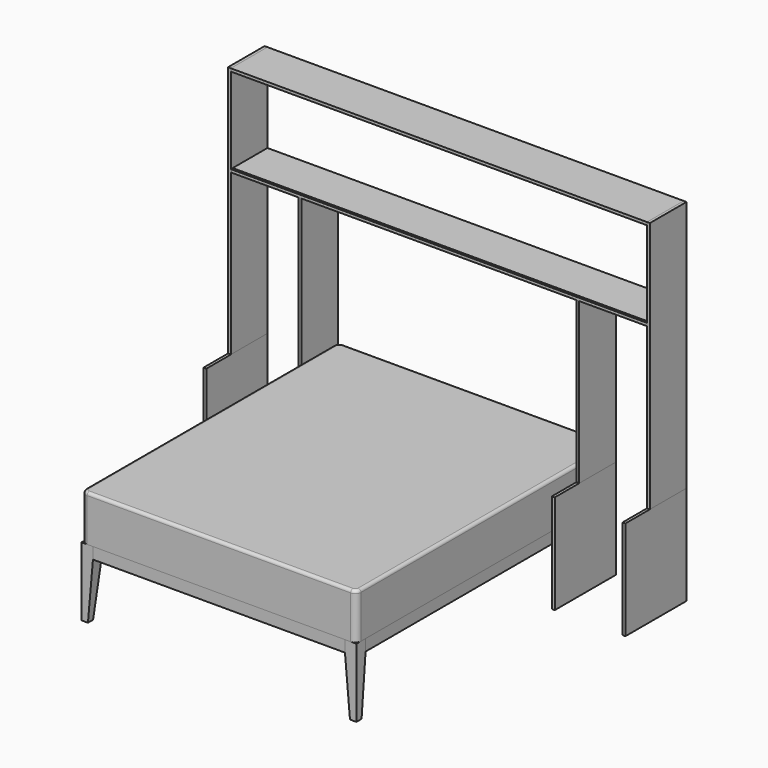
from build123d import *

# Parameters (mm, degrees)
F0_W      = 1828.8
F0_H      = 2133.6
F1_DEPTH  = 304.8
F2_R      = 38.1
F3_R      = 19.05
F5_W      = 76.2
F5_H      = 76.2
F6_DEPTH  = 457.2
F7_SIZE2  = 33.3331808034
F7_SIZE   = 381
F9_DEPTH  = 1676.4
F10_DEPTH = 2057.4
F11_W     = 508
F11_H     = 660.4
F12_DEPTH = 19.05
F15_W     = 19.05
F15_H     = 304.8
F16_DEPTH = 1676.4
F17_DEPTH = 1066.8
F20_DEPTH = 2768.6


with BuildPart() as f1:
    # F0 (on Top) → F1 (new body)
    with BuildSketch(Plane.XY):
        Rectangle(F0_W, F0_H)
    extrude(amount=F1_DEPTH)

    # F2
    f2_edges = [f1.edges().sort_by_distance(p)[0] for p in [
        (-914.4, -1066.8, 152.4),
        (914.4, -1066.8, 152.4),
        (914.4, 1066.8, 152.4),
        (-914.4, 1066.8, 152.4),
    ]]
    fillet(f2_edges, radius=F2_R)

    # F3
    f3_edges = [f1.edges().sort_by_distance(p)[0] for p in [
        (914.4, 0, 304.8),
        (903.240768, -1055.640768, 304.8),
        (903.240768, 1055.640768, 304.8),
        (0, -1066.8, 304.8),
        (0, 1066.8, 304.8),
        (-903.240768, -1055.640768, 304.8),
        (-903.240768, 1055.640768, 304.8),
        (-914.4, 0, 304.8),
    ]]
    fillet(f3_edges, radius=F3_R)


with BuildPart() as f6:
    # F5 (on face) → F6 (new body)
    with BuildSketch(Plane(origin=(0, 0, 0), x_dir=(1, 0, 0), z_dir=(0, 0, -1))):
        with Locations((-876.3, 1028.7)):
            Rectangle(F5_W, F5_H)
    extrude(amount=F6_DEPTH)

    # F7
    f7_edges = [f6.edges().sort_by_distance(p)[0] for p in [
        (-876.3, -990.6, -457.2),
        (-838.2, -1028.7, -457.2),
    ]]
    chamfer(f7_edges, length=F7_SIZE, length2=F7_SIZE2)


with BuildPart() as f8_1:
    # F8: instance of F6
    add(f6.part.mirror(Plane.YZ))


with BuildPart() as f9:
    # F9 (new, through all): a face of the model
    f9_faces = [f6.part.faces().sort_by_distance(p)[0] for p in [
        (-838.2, -1028.7, -38.1),
    ]]
    extrude(f9_faces, amount=F9_DEPTH)


with BuildPart() as f10:
    # F10 (new, through all): a face of the model
    f10_faces = [f8_1.part.faces().sort_by_distance(p)[0] for p in [
        (876.3, -990.6, -38.1),
    ]]
    extrude(f10_faces, amount=F10_DEPTH)


with BuildPart() as f10b:
    # F10#2 (new, through all): a face of the model
    f10_2_faces = [f6.part.faces().sort_by_distance(p)[0] for p in [
        (-876.3, -990.6, -38.1),
    ]]
    extrude(f10_2_faces, amount=F10_DEPTH)


with BuildPart() as f12:
    # F11 (on face) → F12 (new body)
    with BuildSketch(Plane.YZ.offset(914.4)):
        with Locations((812.8, -127)):
            Rectangle(F11_W, F11_H)
    extrude(amount=F12_DEPTH)


with BuildPart() as f14_1:
    # F14: instance of F12
    add(f12.part.mirror(Plane(origin=(1158.875, 812.8, -127), x_dir=(0, 1, 0), z_dir=(1, 0, 0))))


with BuildPart() as f16:
    # F15 (on face) → F16 (new body)
    with BuildSketch(Plane.XY.offset(203.2)):
        with Locations((1393.825, 914.4)):
            Rectangle(F15_W, F15_H)
    extrude(amount=F16_DEPTH)


with BuildPart() as f17:
    # F15 (on face) → F17 (new body, through all)
    with BuildSketch(Plane.XY.offset(203.2)):
        with Locations((923.925, 914.4)):
            Rectangle(F15_W, F15_H)
    extrude(amount=F17_DEPTH)


with BuildPart() as f18_1:
    # F18: instance of F12
    add(f12.part.mirror(Plane.YZ))


with BuildPart() as f18_2:
    # F18: instance of F16
    add(f16.part.mirror(Plane.YZ))


with BuildPart() as f18_3:
    # F18: instance of F14_1
    add(f14_1.part.mirror(Plane.YZ))


with BuildPart() as f18_4:
    # F18: instance of F17
    add(f17.part.mirror(Plane.YZ))


with BuildPart() as f20:
    # F19 (on face) → F20 (new body, through all)
    with BuildSketch(Plane(origin=(1384.3, 0, 0), x_dir=(0, -1, 0), z_dir=(-1, 0, 0))):
        Polygon((-762, 1879.6), (-1066.8, 1879.6), (-1066.8, 1860.55), (-777.875, 1860.55), (-777.875, 1866.9), (-774.7, 1866.9), (-774.7, 1860.55), (-771.525, 1860.55), (-771.525, 1866.9), (-768.35, 1866.9), (-768.35, 1860.55), (-762, 1860.55), align=None)
    extrude(amount=F20_DEPTH)


with BuildPart() as f20b:
    # F19 (on face) → F20, piece 2 (new body, through all)
    with BuildSketch(Plane(origin=(1384.3, 0, 0), x_dir=(0, -1, 0), z_dir=(-1, 0, 0))):
        Polygon((-777.875, 1289.05), (-1066.8, 1289.05), (-1066.8, 1270), (-762, 1270), (-762, 1289.05), (-768.35, 1289.05), (-768.35, 1285.875), (-771.525, 1285.875), (-771.525, 1289.05), (-774.7, 1289.05), (-774.7, 1285.875), (-777.875, 1285.875), align=None)
    extrude(amount=F20_DEPTH)


solid = Compound([f1.part, f6.part, f8_1.part, f9.part, f10.part, f10b.part, f12.part, f14_1.part, f16.part, f17.part, f18_1.part, f18_2.part, f18_3.part, f18_4.part, f20.part, f20b.part])
